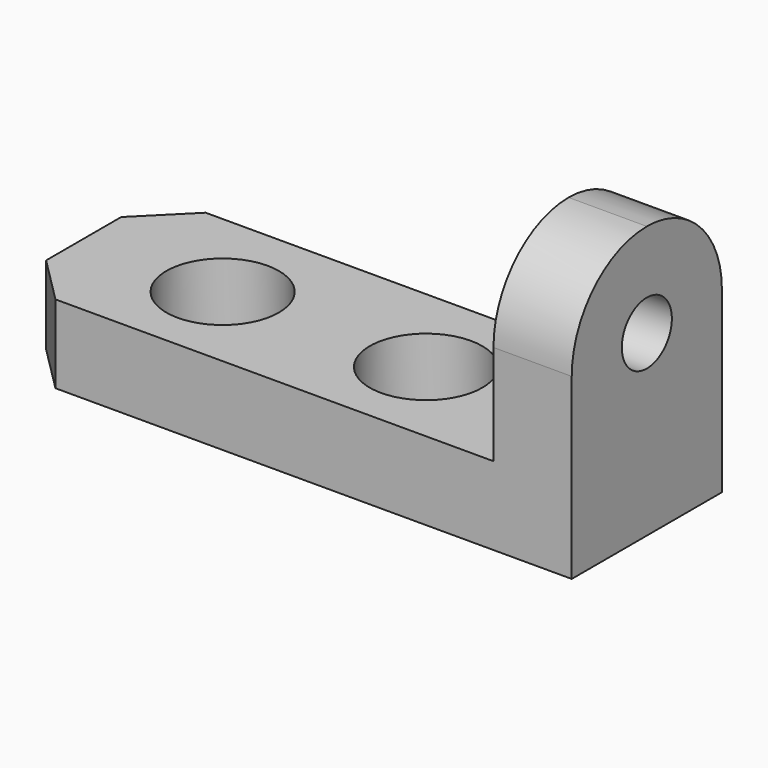
from build123d import *

# Parameters (mm, degrees)
F0_W     = 4572
F0_H     = 1524
F1_DEPTH = 635
F2_W     = 635.3021987379
F2_H     = 1524
F3_DEPTH = 1574.8
F4_R     = 761.99999
F5_R     = 457.2
F6_DEPTH = 889
F7_R     = 254
F8_DEPTH = 635
F9_DEPTH = 25.4
F10_SIZE = 381


# Not quite as in the source:
# - a fillet or chamfer is up to 0.001 mm smaller than in the source, because OpenCascade refuses the exact size


with BuildPart() as f1:
    # F0 (on Top) → F1 (new body)
    with BuildSketch(Plane.XY):
        with Locations((-1.0364986956, 18.1390648085)):
            Rectangle(F0_W, F0_H)
    extrude(amount=F1_DEPTH)

    # F2 (on face) → F3 (join)
    with BuildSketch(Plane.XY.offset(635)):
        with Locations((1967.3124019355, 18.1390648085)):
            Rectangle(F2_W, F2_H)
    extrude(amount=F3_DEPTH)

    # F4 (radius 762 in the source; OpenCascade refuses exactly that, so slightly less here)
    f4_edges = [f1.edges().sort_by_distance(p)[0] for p in [
        (1967.312402, 780.139065, 2209.8),
        (1967.312402, -743.860935, 2209.8),
    ]]
    fillet(f4_edges, radius=F4_R)

    # F5 (on face) → F6 (cut)
    with BuildSketch(Plane.XY.offset(635)):
        with Locations((-1144.0364986956, 0)):
            Circle(F5_R)
        with Locations((506.9635013044, 0)):
            Circle(F5_R)
    extrude(amount=-F6_DEPTH, mode=Mode.SUBTRACT)

    # F7 (on face) → F8 (cut)
    with BuildSketch(Plane(origin=(1649.6613025665, 0, 0), x_dir=(0, -1, 0), z_dir=(-1, 0, 0))):
        with Locations((-18.1390648085, 1447.8)):
            Circle(F7_R)
    extrude(amount=-F8_DEPTH, mode=Mode.SUBTRACT)

    # F9 (cut): a face of the model
    f9_faces = [f1.faces().sort_by_distance(p)[0] for p in [
        (2284.6613025665, 18.1390648085, 1447.8),
    ]]
    extrude(f9_faces, amount=-F9_DEPTH, mode=Mode.SUBTRACT)

    # F10
    f10_edges = [f1.edges().sort_by_distance(p)[0] for p in [
        (-2287.036499, -743.860935, 317.5),
        (-2287.036499, 780.139065, 317.5),
    ]]
    chamfer(f10_edges, length=F10_SIZE)


solid = f1.part
